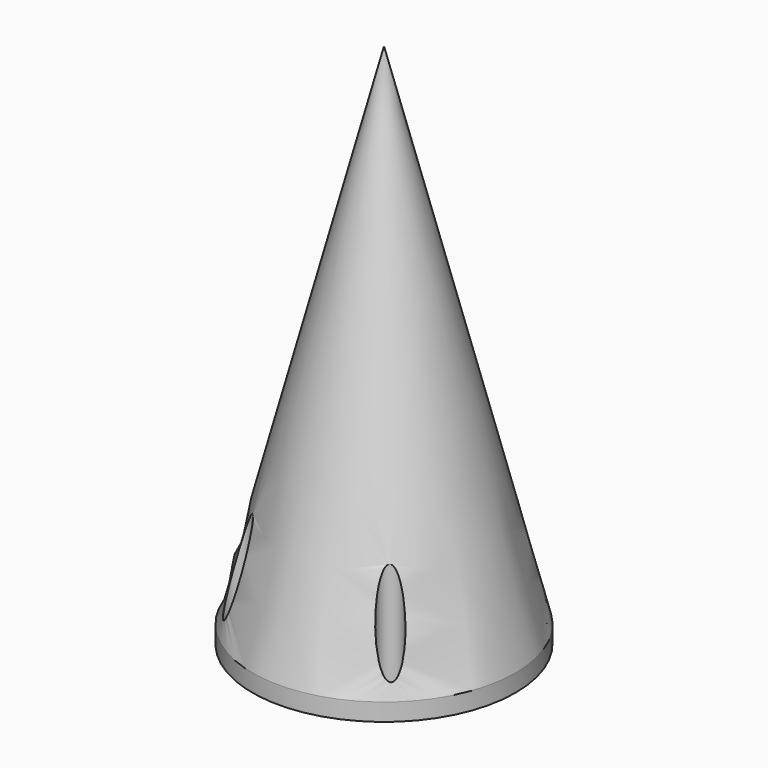
from build123d import *

# Parameters (mm, degrees)
F0_R           = 25
F1_DEPTH       = 100
F3_D           = 2.5
F3_CBORE_D     = 4.5
F3_CBORE_DEPTH = 98
F5_T           = 5


# Not quite as in the source:
# - a fillet or chamfer that OpenCascade refuses, or shapes differently, is made with other operations: its cross-section is extruded or revolved along the edge and cut away or added
# - a shell that OpenCascade refuses in one call is made with other operations: the cavity is built on its own and cut out


with BuildPart() as f1:
    # F0 (on Top) → F1 (new body)
    with BuildSketch(Plane.XY):
        Circle(F0_R)
    extrude(amount=F1_DEPTH)

    # F3 (through all)
    with Locations(Plane.XY.offset(100)):
        with Locations((14.4662138687, 16.5749406124), (14.4662138687, -16.5749406124), (-14.4662138687, -16.5749406124), (-14.4662138687, 16.5749406124)):
            CounterBoreHole(F3_D / 2, F3_CBORE_D / 2, F3_CBORE_DEPTH)

    # F4: chamfer of 25 x 96.6678273725 on 1 edges, made by hand

    # F4_s1 → F4_t2 (revolve, cut)
    with BuildSketch(Plane.XZ):
        Polygon((25, 3.3321726275), (0, 100), (25, 100), align=None)
    revolve(axis=Axis((0, 0, 100), (0, 0, 1)), mode=Mode.SUBTRACT)

    # F5: shell of thickness 5, made by hand


with BuildPart() as f5_core1:
    # F5_t2: copy of F1
    add(f1.part)

    # the walls: a layer under each face that stays
    f5_faces = [f5_core1.faces().sort_by_distance(p)[0] for p in [
        (-25, 0, 1.6660863138),
        (-12.5, 0, 51.6660863138),
        (-15.7162138687, -16.5749406124, 1),
        (13.2162138687, -16.5749406124, 1),
        (-15.7162138687, 16.5749406124, 1),
        (13.2162138687, 16.5749406124, 1),
        (12.2162138687, 16.5749406124, 12.8162373482),
        (-13.3412138687, -14.6263834539, 5.6054124494),
        (-13.3412138687, 18.523497771, 5.6054156171),
        (12.2162138687, -16.5749406124, 12.8162468512),
        (-15.9662138687, -18.0749406124, 2),
        (12.9662138687, -18.0749406124, 2),
        (-15.9662138687, 15.0749406124, 2),
        (12.9662138687, 15.0749406124, 2),
    ]]
    thicken(f5_faces, amount=-F5_T, mode=Mode.SUBTRACT)

    # F5_s3 → F5_t4 (revolve, cut)
    with BuildSketch(Plane.XZ.offset(-16.5749406124)):
        Polygon((16.6662138687, 2.05), (21.7162138687, 2), (21.7162138687, -3), (16.7162138687, -3), align=None)
    revolve(axis=Axis((14.4662138687, 16.5749406124, 2), (0, 0, 1)), mode=Mode.SUBTRACT)

    # F5_s5 → F5_t6 (revolve, cut)
    with BuildSketch(Plane.XZ.offset(16.5749406124)):
        Polygon((-12.2662138687, 2.05), (-7.2162138687, 2), (-7.2162138687, -3), (-12.2162138687, -3), align=None)
    revolve(axis=Axis((-14.4662138687, -16.5749406124, 2), (0, 0, 1)), mode=Mode.SUBTRACT)

    # F5_s7 → F5_t8 (revolve, cut)
    with BuildSketch(Plane.XZ.offset(-16.5749406124)):
        Polygon((-12.2662138687, 2.05), (-7.2162138687, 2), (-7.2162138687, -3), (-12.2162138687, -3), align=None)
    revolve(axis=Axis((-14.4662138687, 16.5749406124, 2), (0, 0, 1)), mode=Mode.SUBTRACT)

    # F5_s9 → F5_t10 (revolve, cut)
    with BuildSketch(Plane.XZ.offset(16.5749406124)):
        Polygon((16.6662138687, 2.05), (21.7162138687, 2), (21.7162138687, -3), (16.7162138687, -3), align=None)
    revolve(axis=Axis((14.4662138687, -16.5749406124, 2), (0, 0, 1)), mode=Mode.SUBTRACT)


with BuildPart() as f1_1:
    add(f1.part)

    # what is left inside the walls is the cavity
    f5_cavity = [f5_core1.part.solids().sort_by_distance(p)[0] for p in [
        (-13.284926, 0, 28.461661),
    ]]
    add(f5_cavity, mode=Mode.SUBTRACT)


solid = f1_1.part
